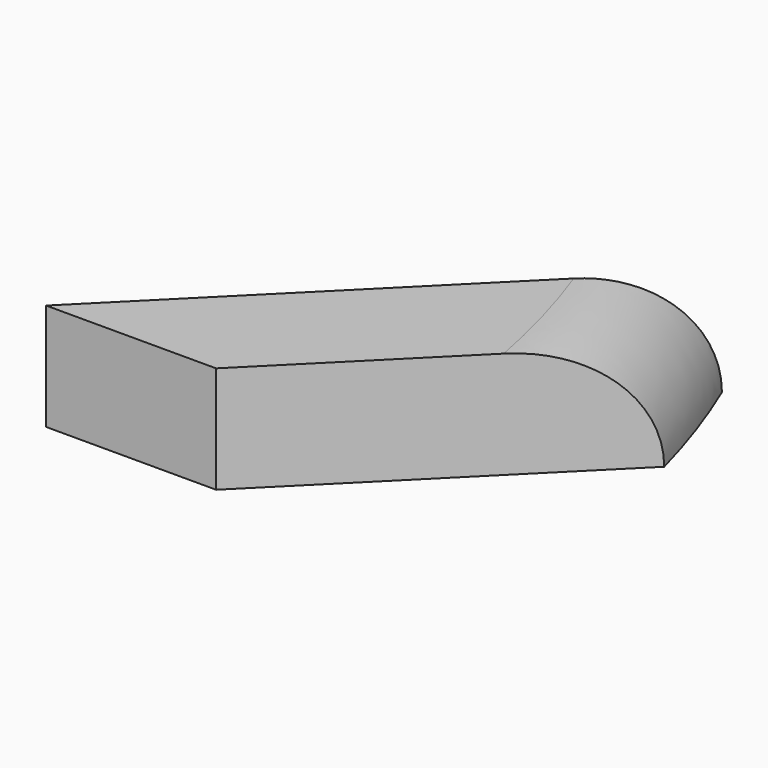
from build123d import *

# Parameters (mm, degrees)
F2_DEPTH = 25.4
F3_R     = 25.39999


# Not quite as in the source:
# - a fillet or chamfer is up to 0.001 mm smaller than in the source, because OpenCascade refuses the exact size


with BuildPart() as f2:
    # F1 (on face) → F2 (new body)
    with BuildSketch(Plane.XY):
        with BuildLine():
            Line((210.4652929995, 89.2318353651), (121.2334576344, 0))
            Line((121.2334576344, 0), (161.6446101792, 0))
            Line((161.6446101792, 0), (220.8106438897, 59.1660337104))
            ThreePointArc((220.8106438897, 59.1660337104), (216.1613322086, 74.3790189354), (210.4652929995, 89.2318353651))
        make_face()
    extrude(amount=F2_DEPTH)

    # F3 (radius 25.4 in the source; OpenCascade refuses exactly that, so slightly less here)
    f3_edges = [f2.edges().sort_by_distance(p)[0] for p in [
        (216.161332, 74.379019, 25.4),
    ]]
    fillet(f3_edges, radius=F3_R)


solid = f2.part
